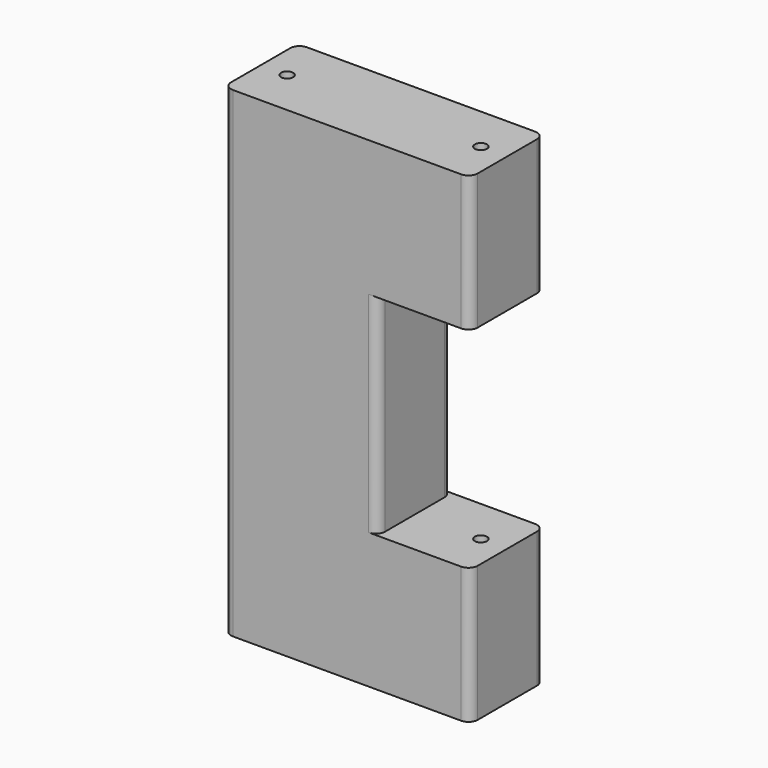
from build123d import *

# Parameters (mm, degrees)
F0_W     = 6.35
F0_H     = 8.636
F1_DEPTH = 3.81
F3_START = -0.000254
F3_DEPTH = 3.81
F4_R     = 0.2501042953
F5_DEPTH = 50.8
F6_R     = 0.381


# Not quite as in the source:
# - a feature names something its author has since deleted; it is built from what else it names


with BuildPart() as f1:
    # F0 (on Front) → F1 (new body)
    with BuildSketch(Plane.XZ):
        Polygon((27.1829397243, -29.1464989846), (17.0229397243, -29.1464989846), (17.0229397243, -34.7344989846), (23.3729397243, -34.7344989846), (27.1829397243, -34.7344989846), align=None)
        with Locations((20.1979397243, -39.0524989846)):
            Rectangle(F0_W, F0_H)
        Polygon((23.3729397243, -43.3704989846), (17.0229397243, -43.3704989846), (17.0229397243, -48.9584989846), (23.3729397243, -48.9584989846), (27.1829397243, -48.9584989846), (27.1829397243, -43.3704989846), align=None)
    extrude(amount=F1_DEPTH)

    # F2 (on face) → F3 (join)
    with BuildSketch(Plane.XZ.offset(3.81).offset(F3_START)):
        Polygon((27.1829397243, -29.1464989846), (17.0229397243, -29.1464989846), (17.0229397243, -34.7344989846), (23.3729397243, -34.7344989846), (27.1829397243, -34.7344989846), align=None)
        Polygon((27.1829397243, -43.3704989846), (23.3729397243, -43.3704989846), (17.0229397243, -43.3704989846), (17.0229397243, -48.9584989846), (27.1829397243, -48.9584989846), align=None)
    extrude(amount=-F3_DEPTH)

    # F4 (on face) → F5 (cut)
    with BuildSketch(Plane(origin=(0, 0, -48.9584989846), x_dir=(1, 0, 0), z_dir=(0, 0, -1))):
        with Locations((26.094635429, 1.904746)):
            Circle(F4_R)
        with Locations((18.1112440196, 1.904746)):
            Circle(F4_R)
    extrude(amount=-F5_DEPTH, mode=Mode.SUBTRACT)

    # F6 (call 1 of 10: OpenCascade refuses the feature's edges together)
    f6_edges = [f1.edges().sort_by_distance(p)[0] for p in [
        (27.18294, -3.81, -31.940499),
    ]]
    fillet(f6_edges, radius=F6_R)

    # F6#2 (call 2 of 10)
    f6_2_edges = [f1.edges().sort_by_distance(p)[0] for p in [
        (17.02294, -3.81, -39.052499),
    ]]
    fillet(f6_2_edges, radius=F6_R)

    # F6#3 (call 3 of 10)
    f6_3_edges = [f1.edges().sort_by_distance(p)[0] for p in [
        (27.18294, -3.81, -46.164499),
    ]]
    fillet(f6_3_edges, radius=F6_R)

    # F6#4 (call 4 of 10)
    f6_4_edges = [f1.edges().sort_by_distance(p)[0] for p in [
        (23.37294, -3.81, -39.052499),
    ]]
    fillet(f6_4_edges, radius=F6_R)

    # F6#5 (call 5 of 10)
    f6_5_edges = [f1.edges().sort_by_distance(p)[0] for p in [
        (23.37294, 0, -39.052499),
    ]]
    fillet(f6_5_edges, radius=F6_R)

    # F6#7 (call 6 of 10)
    f6_7_edges = [f1.edges().sort_by_distance(p)[0] for p in [
        (27.18294, 0.000254, -31.940499),
    ]]
    fillet(f6_7_edges, radius=F6_R)

    # F6#8 (call 7 of 10)
    f6_8_edges = [f1.edges().sort_by_distance(p)[0] for p in [
        (27.18294, 0.000254, -46.164499),
    ]]
    fillet(f6_8_edges, radius=F6_R)

    # F6#10 (call 8 of 10)
    f6_10_edges = [f1.edges().sort_by_distance(p)[0] for p in [
        (17.02294, 0, -39.052499),
    ]]
    fillet(f6_10_edges, radius=F6_R)

    # F6#6 (call 9 of 10)
    f6_6_edges = [f1.edges().sort_by_distance(p)[0] for p in [
        (17.02294, 0.000254, -31.940499),
    ]]
    fillet(f6_6_edges, radius=F6_R)

    # F6#9 (call 10 of 10)
    f6_9_edges = [f1.edges().sort_by_distance(p)[0] for p in [
        (17.02294, 0.000254, -46.164499),
    ]]
    fillet(f6_9_edges, radius=F6_R)


solid = f1.part
